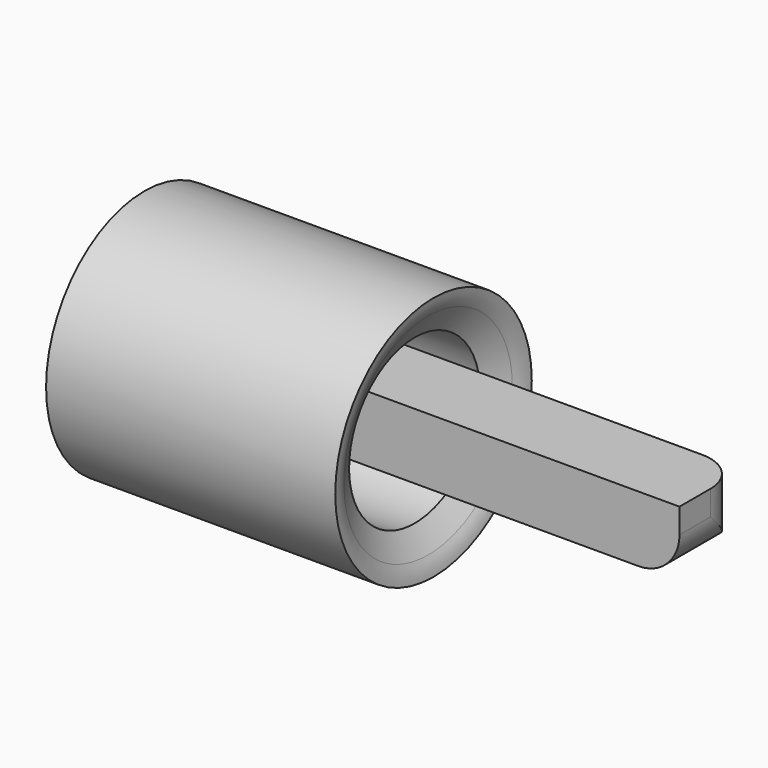
from build123d import *

# Parameters (mm, degrees)
F3_W     = 9.723054
F3_H     = 8.02152
F4_DEPTH = 50
F5_R     = 5


# Not quite as in the source:
# - a fillet or chamfer that OpenCascade refuses, or shapes differently, is made with other operations: its cross-section is extruded or revolved along the edge and cut away or added


with BuildPart() as f1:
    # F0 (on Front) → F1 (revolve)
    with BuildSketch(Plane.XZ):
        Polygon((-16, 4), (-4, 4), (0, 0), (2, 0), (2, 10), (17, 10), (19.309401, 14), (19.309401, 15), (-13.687211, 15), (-16, 15), align=None)
    revolve(axis=Axis((0.643679, 0, 0), (1, 0, 0)))

    # F2: fillet of radius 5 on 1 edges, made by hand

    # F2_s1 → F2_t2 (revolve, cut)
    with BuildSketch(Plane.XZ):
        with BuildLine():
            ThreePointArc((19.309401, 15), (19.102065, 13.894089), (18.652689, 12.862541))
            Line((18.652689, 12.862541), (18.739292, 12.812541))
            Line((18.739292, 12.812541), (19.396004, 13.95))
            Line((19.396004, 13.95), (19.409401, 14))
            ThreePointArc((19.409401, 14), (19.409401, 14.5), (19.409138, 14.992749))
            Line((19.409138, 14.992749), (19.309401, 15))
        make_face()
    revolve(axis=Axis((19.309401, 0, 0), (1, 0, 0)), mode=Mode.SUBTRACT)

    # F3 (on face) → F4 (join)
    with BuildSketch(Plane.YZ.offset(2)):
        with Locations((1.542801, 0.525098)):
            Rectangle(F3_W, F3_H)
    extrude(amount=F4_DEPTH)

    # F5
    f5_edges = [f1.edges().sort_by_distance(p)[0] for p in [
        (52, 1.542801, -3.485662),
        (52, 6.404328, 0.525098),
    ]]
    fillet(f5_edges, radius=F5_R)


solid = f1.part
